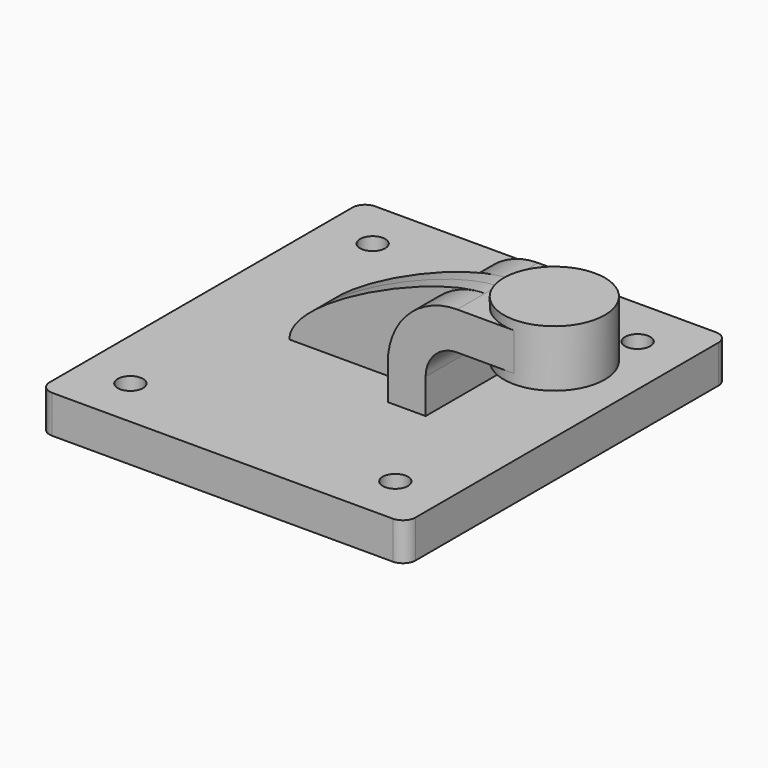
from build123d import *

# Parameters (mm, degrees)
F1_DEPTH = 101.6
F0_W     = 25.4
F0_H     = 19.05
F2_DEPTH = 25.4
F3_DEPTH = 7.9375
F5_R     = 6.35
F6_R     = 6.35
F7_DEPTH = 19.051


# Not quite as in the source:
# - a feature names something its author has since deleted; it is built from what else it names


with BuildPart() as f1:
    # F0 (on Front) → F1 (new body, symmetric)
    with BuildSketch(Plane.XZ):
        Polygon((-92.075, -9.525), (-41.275, -9.525), (41.275, -9.525), (92.075, -9.525), (92.075, 9.525), (41.275, 9.525), (22.225, 9.525), (-41.275, 9.525), (-92.075, 9.525), align=None)
    extrude(amount=F1_DEPTH, both=True)

    # F0 (on Front) → F2 (join, symmetric)
    with BuildSketch(Plane.XZ):
        with BuildLine():
            Line((22.225, 9.525), (41.275, 9.525))
            Line((41.275, 9.525), (41.275, 27.0002))
            ThreePointArc((41.275, 27.0002), (45.9246798487, 38.2255201513), (57.15, 42.8752))
            Line((57.15, 42.8752), (60.325, 42.8752))
            Line((60.325, 42.8752), (60.325, 61.9252))
            Line((60.325, 61.9252), (57.15, 61.9252))
            ThreePointArc((57.15, 61.9252), (32.4542956671, 51.6959043329), (22.225, 27.0002))
            Line((22.225, 27.0002), (22.225, 9.525))
        make_face()
        with Locations((73.025, 52.4002)):
            Rectangle(F0_W, F0_H)
    extrude(amount=F2_DEPTH, both=True)

    # F0 (on Front) → F3 (join, symmetric)
    with BuildSketch(Plane.XZ):
        with BuildLine():
            add(Edge.make_bspline(
                [(-41.275, 9.525), (-41.1597527564, 29.4812973589), (32.6236560941, 62.2739233077), (57.15, 61.9252)],
                knots=[0, 0, 0, 0, 111.5045361635, 111.5045361635, 111.5045361635, 111.5045361635], degree=3))
            Line((-41.275, 9.525), (22.225, 9.525))
            Line((22.225, 9.525), (22.225, 27.0002))
            ThreePointArc((22.225, 27.0002), (32.4542956671, 51.6959043329), (57.15, 61.9252))
        make_face()
    extrude(amount=F3_DEPTH, both=True)

    # F0 (on Front) → F4 (revolve)
    with BuildSketch(Plane.XZ):
        Polygon((85.725, 66.675), (85.725, 61.9252), (85.725, 42.8752), (85.725, 38.1), (111.125, 38.1), (111.125, 66.675), align=None)
    revolve(axis=Axis((85.725, 0, 52.3875), (0, 0, 1)))

    # F5
    f5_edges = [f1.edges().sort_by_distance(p)[0] for p in [
        (-92.075, -101.6, 0),
        (92.075, -101.6, 0),
        (92.075, 101.6, 0),
        (-92.075, 101.6, 0),
    ]]
    fillet(f5_edges, radius=F5_R)

    # F6 (on face) → F7 (cut, through all)
    with BuildSketch(Plane.XY.offset(9.525)):
        with Locations((66.675, 76.2)):
            Circle(F6_R)
        with Locations((66.675, -76.2)):
            Circle(F6_R)
        with Locations((-66.675, 76.2)):
            Circle(F6_R)
        with Locations((-66.675, -76.2)):
            Circle(F6_R)
    extrude(amount=-F7_DEPTH, mode=Mode.SUBTRACT)


solid = f1.part
